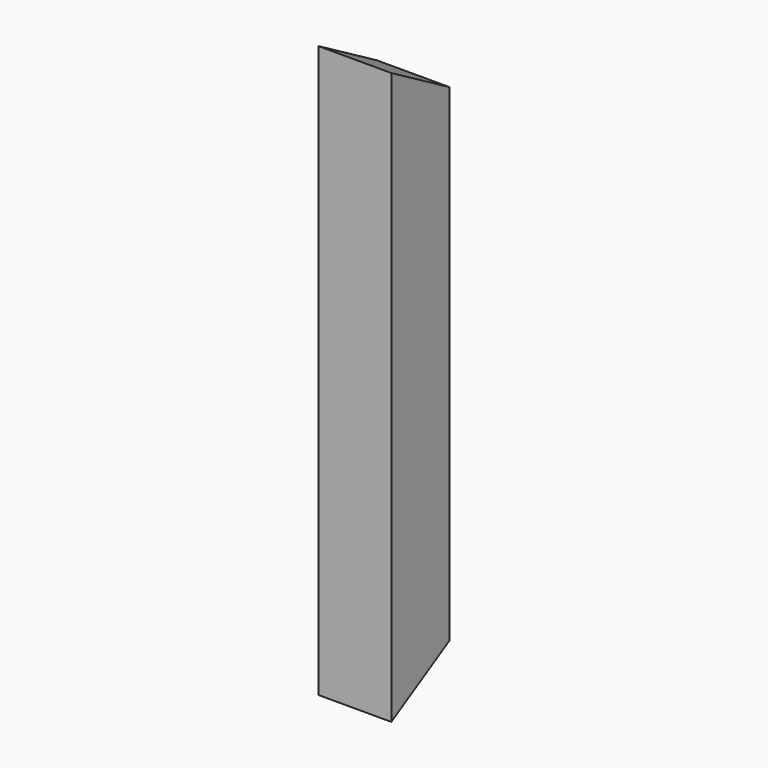
from build123d import *

# Parameters (mm, degrees)
F0_W     = 150
F0_H     = 150
F1_DEPTH = 587.5
F3_DEPTH = 150


# Not quite as in the source:
# - a pattern or mirror of a feature is missing from the dataset's text; its kind, count and spacing are read off the source's solid


with BuildPart() as f1:
    # F0 (on Top) → F1 (new body, symmetric)
    with BuildSketch(Plane.XY):
        Rectangle(F0_W, F0_H)
    extrude(amount=F1_DEPTH, both=True)

    # F2 (on face) → F3 (cut, through all)
    with BuildSketch(Plane.YZ.offset(75)):
        Polygon((75, 587.5), (-75, 587.5), (75, 500.8974596216), align=None)
    f3 = extrude(amount=-F3_DEPTH, mode=Mode.SUBTRACT)

    # F3_copies: F3 across plane
    add(f3.mirror(Plane(origin=(0, 0, 0), x_dir=(-1, 0, 0), z_dir=(0, 0, -1))), mode=Mode.SUBTRACT)


solid = f1.part
